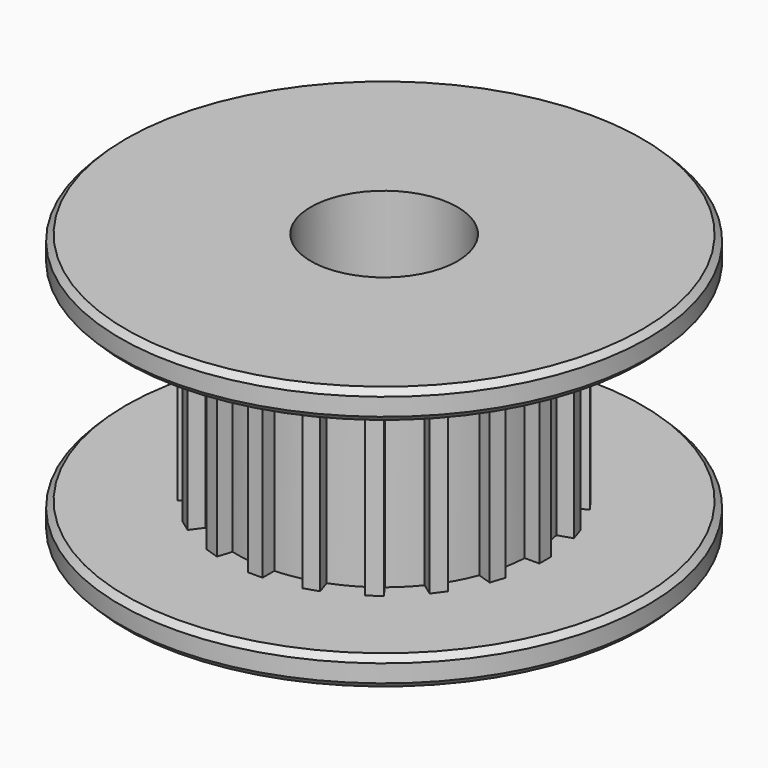
from build123d import *

# Parameters (mm, degrees)
F3_DEPTH        = 7
F3_COPIES_COUNT = 20
F4_SIZE         = 0.2


# Not quite as in the source:
# - a pattern or mirror of a feature is missing from the dataset's text; its kind, count and spacing are read off the source's solid


with BuildPart() as f1:
    # F0 (on Front) → F1 (revolve)
    with BuildSketch(Plane.XZ):
        Polygon((2.5, 9), (2.5, 0), (9, 0), (9, 1), (5, 1), (5, 8), (9, 8), (9, 9), align=None)
    revolve(axis=Axis((0, 0, 4.5), (0, 0, -1)))

    # F2 (on face) → F3 (join, through all)
    with BuildSketch(Plane.XY.offset(1)):
        with BuildLine():
            Line((-0.25, 5.4937460889), (-0.25, 4.9937460889))
            ThreePointArc((-0.25, 4.9937460889), (0, 5), (0.25, 4.9937460889))
            Line((0.25, 4.9937460889), (0.25, 5.4937460889))
            Line((0.25, 5.4937460889), (-0.25, 5.4937460889))
        make_face()
    f3 = extrude(amount=F3_DEPTH)

    # F3_copies: F3 ×20 about axis
    f3_copies_axis = Axis((0, 0, 0), (0, 0, 1))
    for i in range(1, F3_COPIES_COUNT):
        add(f3.rotate(f3_copies_axis, i * 360 / F3_COPIES_COUNT))

    # F4
    f4_edges = [f1.edges().sort_by_distance(p)[0] for p in [
        (-9, 0, 9),
        (-9, 0, 8),
        (-9, 0, 1),
        (-9, 0, 0),
    ]]
    chamfer(f4_edges, length=F4_SIZE)


solid = f1.part
